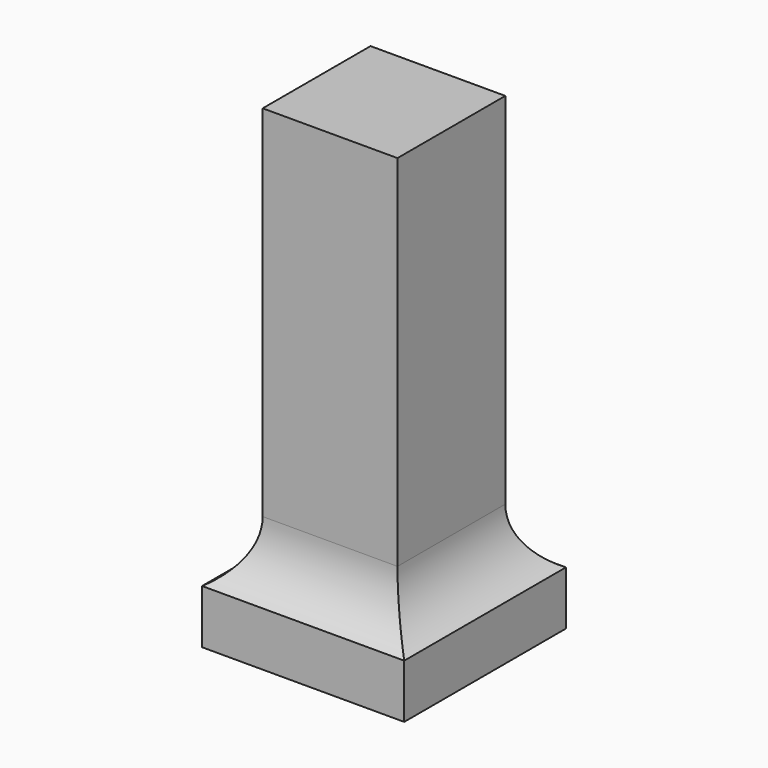
from build123d import *

# Parameters (mm, degrees)
F0_W         = 10
F0_H         = 10
F1_DEPTH     = 35
F2_W         = 15
F2_H         = 15
F3_DEPTH     = 4
F4_T1_DEPTH  = 10
F4_T3_DEPTH  = 10
F4_T9_DEPTH  = 20.8253175473
F4_T14_DEPTH = 20.8253175473
F4_T22_DEPTH = 20.8253175473
F4_T27_DEPTH = 20.8253175473
F4_T35_DEPTH = 20.8253175473
F4_T40_DEPTH = 20.8253175473
F4_T48_DEPTH = 20.8253175473
F4_T53_DEPTH = 20.8253175473


# Not quite as in the source:
# - a fillet or chamfer that OpenCascade refuses, or shapes differently, is made with other operations: its cross-section is extruded or revolved along the edge and cut away or added


with BuildPart() as f1:
    # F0 (on Top) → F1 (new body)
    with BuildSketch(Plane.XY):
        Rectangle(F0_W, F0_H)
    extrude(amount=F1_DEPTH)

    # F2 (on Top) → F3 (join)
    with BuildSketch(Plane.XY):
        Rectangle(F2_W, F2_H)
    extrude(amount=F3_DEPTH)

    # F4: fillet of radius 5 on 4 edges, made by hand

    # F4_s2 → F4_t1 (join)
    with BuildSketch(Plane.XZ.offset(-5)):
        with BuildLine():
            ThreePointArc((-7.5, 4), (-5.6698729811, 5.8301270189), (-5, 8.3301270189))
            Line((-5, 8.3301270189), (-5, 4))
            Line((-5, 4), (-7.5, 4))
        make_face()
        with BuildLine():
            ThreePointArc((7.5, 4), (5.6698729811, 5.8301270189), (5, 8.3301270189))
            Line((5, 8.3301270189), (5, 4))
            Line((5, 4), (7.5, 4))
        make_face()
    extrude(amount=F4_T1_DEPTH)

    # F4_s4 → F4_t3 (join)
    with BuildSketch(Plane.YZ.offset(-5)):
        with BuildLine():
            ThreePointArc((7.5, 4), (5.6698729811, 5.8301270189), (5, 8.3301270189))
            Line((5, 8.3301270189), (5, 4))
            Line((5, 4), (7.5, 4))
        make_face()
        with BuildLine():
            ThreePointArc((-7.5, 4), (-5.6698729811, 5.8301270189), (-5, 8.3301270189))
            Line((-5, 8.3301270189), (-5, 4))
            Line((-5, 4), (-7.5, 4))
        make_face()
    extrude(amount=F4_T3_DEPTH)


with BuildPart() as f4_tool7:
    # F4_s8 → F4_t9 (new body)
    with BuildSketch(Plane.YZ.offset(5)):
        with BuildLine():
            ThreePointArc((7.5, 4), (5.6698729811, 5.8301270189), (5, 8.3301270189))
            Line((5, 8.3301270189), (5, 4))
            Line((5, 4), (7.5, 4))
        make_face()
    extrude(amount=-F4_T9_DEPTH)

    split(bisect_by=Plane.YZ.offset(-7.5), keep=Keep.TOP)

    split(bisect_by=Plane.YZ.offset(-5), keep=Keep.BOTTOM)


with BuildPart() as f4_tool12:
    # F4_s13 → F4_t14 (new body)
    with BuildSketch(Plane.XZ.offset(-15.8253175473)):
        with BuildLine():
            ThreePointArc((-7.5, 4), (-5.6698729811, 5.8301270189), (-5, 8.3301270189))
            Line((-5, 8.3301270189), (-5, 4))
            Line((-5, 4), (-7.5, 4))
        make_face()
    extrude(amount=F4_T14_DEPTH)

    split(bisect_by=Plane.XZ.offset(-7.5), keep=Keep.TOP)

    split(bisect_by=Plane.XZ.offset(-5), keep=Keep.BOTTOM)


with BuildPart() as f4_tool7_1:
    add(f4_tool7.part)

    # F4_t17: intersect F4_tool12
    add(f4_tool12.part, mode=Mode.INTERSECT)


with BuildPart() as f1_1:
    add(f1.part)

    # F4_t5: union F4_tool7
    add(f4_tool7_1.part)


with BuildPart() as f4_tool20:
    # F4_s21 → F4_t22 (new body)
    with BuildSketch(Plane.XZ.offset(-5)):
        with BuildLine():
            ThreePointArc((-7.5, 4), (-5.6698729811, 5.8301270189), (-5, 8.3301270189))
            Line((-5, 8.3301270189), (-5, 4))
            Line((-5, 4), (-7.5, 4))
        make_face()
    extrude(amount=F4_T22_DEPTH)

    split(bisect_by=Plane.XZ.offset(7.5), keep=Keep.BOTTOM)

    split(bisect_by=Plane.XZ.offset(5), keep=Keep.TOP)


with BuildPart() as f4_tool25:
    # F4_s26 → F4_t27 (new body)
    with BuildSketch(Plane.YZ.offset(-15.8253175473)):
        with BuildLine():
            ThreePointArc((-7.5, 4), (-5.6698729811, 5.8301270189), (-5, 8.3301270189))
            Line((-5, 8.3301270189), (-5, 4))
            Line((-5, 4), (-7.5, 4))
        make_face()
    extrude(amount=F4_T27_DEPTH)

    split(bisect_by=Plane.YZ.offset(-7.5), keep=Keep.TOP)

    split(bisect_by=Plane.YZ.offset(-5), keep=Keep.BOTTOM)


with BuildPart() as f4_tool20_1:
    add(f4_tool20.part)

    # F4_t30: intersect F4_tool25
    add(f4_tool25.part, mode=Mode.INTERSECT)


with BuildPart() as f1_2:
    add(f1_1.part)

    # F4_t18: union F4_tool20
    add(f4_tool20_1.part)


with BuildPart() as f4_tool33:
    # F4_s34 → F4_t35 (new body)
    with BuildSketch(Plane.YZ.offset(15.8253175473)):
        with BuildLine():
            ThreePointArc((7.5, 4), (5.6698729811, 5.8301270189), (5, 8.3301270189))
            Line((5, 8.3301270189), (5, 4))
            Line((5, 4), (7.5, 4))
        make_face()
    extrude(amount=-F4_T35_DEPTH)

    split(bisect_by=Plane.YZ.offset(7.5), keep=Keep.BOTTOM)

    split(bisect_by=Plane.YZ.offset(5), keep=Keep.TOP)


with BuildPart() as f4_tool38:
    # F4_s39 → F4_t40 (new body)
    with BuildSketch(Plane.XZ.offset(5)):
        with BuildLine():
            ThreePointArc((7.5, 4), (5.6698729811, 5.8301270189), (5, 8.3301270189))
            Line((5, 8.3301270189), (5, 4))
            Line((5, 4), (7.5, 4))
        make_face()
    extrude(amount=-F4_T40_DEPTH)

    split(bisect_by=Plane.XZ.offset(-7.5), keep=Keep.TOP)

    split(bisect_by=Plane.XZ.offset(-5), keep=Keep.BOTTOM)


with BuildPart() as f4_tool33_1:
    add(f4_tool33.part)

    # F4_t43: intersect F4_tool38
    add(f4_tool38.part, mode=Mode.INTERSECT)


with BuildPart() as f1_3:
    add(f1_2.part)

    # F4_t31: union F4_tool33
    add(f4_tool33_1.part)


with BuildPart() as f4_tool46:
    # F4_s47 → F4_t48 (new body)
    with BuildSketch(Plane.YZ.offset(-5)):
        with BuildLine():
            ThreePointArc((-7.5, 4), (-5.6698729811, 5.8301270189), (-5, 8.3301270189))
            Line((-5, 8.3301270189), (-5, 4))
            Line((-5, 4), (-7.5, 4))
        make_face()
    extrude(amount=F4_T48_DEPTH)

    split(bisect_by=Plane.YZ.offset(7.5), keep=Keep.BOTTOM)

    split(bisect_by=Plane.YZ.offset(5), keep=Keep.TOP)


with BuildPart() as f4_tool51:
    # F4_s52 → F4_t53 (new body)
    with BuildSketch(Plane.XZ.offset(15.8253175473)):
        with BuildLine():
            ThreePointArc((7.5, 4), (5.6698729811, 5.8301270189), (5, 8.3301270189))
            Line((5, 8.3301270189), (5, 4))
            Line((5, 4), (7.5, 4))
        make_face()
    extrude(amount=-F4_T53_DEPTH)

    split(bisect_by=Plane.XZ.offset(7.5), keep=Keep.BOTTOM)

    split(bisect_by=Plane.XZ.offset(5), keep=Keep.TOP)


with BuildPart() as f4_tool46_1:
    add(f4_tool46.part)

    # F4_t56: intersect F4_tool51
    add(f4_tool51.part, mode=Mode.INTERSECT)


with BuildPart() as f1_4:
    add(f1_3.part)

    # F4_t44: union F4_tool46
    add(f4_tool46_1.part)


solid = f1_4.part
